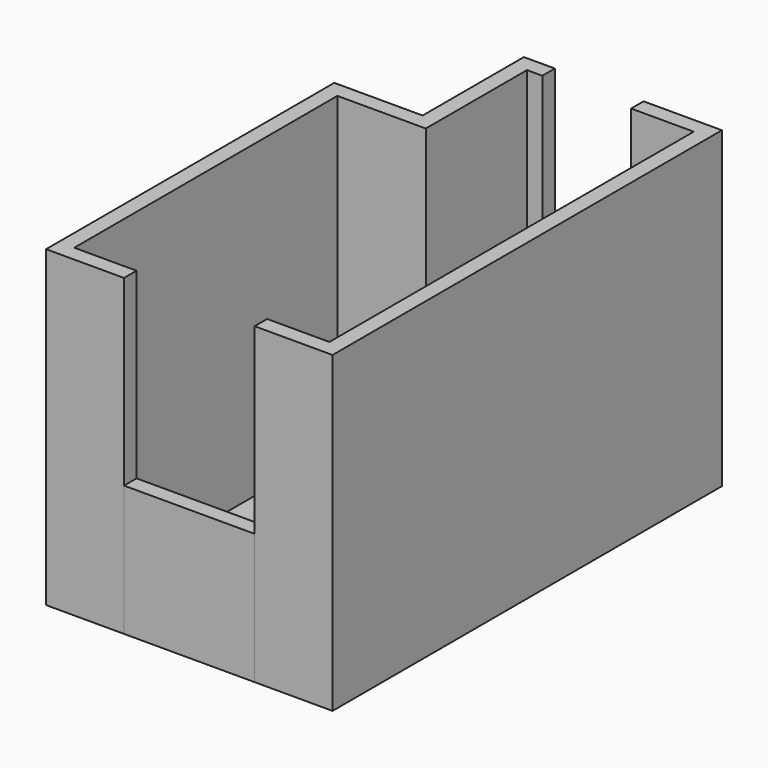
from build123d import *

# Parameters (mm, degrees)
F1_DEPTH = 2400
F0_W     = 1000
F0_H     = 120
F2_DEPTH = 1000
F4_DEPTH = 25


# Not quite as in the source:
# - a feature of the source that left no trace in its solid (it failed there, or was rolled back) is left out


with BuildPart() as f1:
    # F0 (on Top) → F1 (new body)
    with BuildSketch(Plane.XY):
        Polygon((1954, 0), (1477, 0), (1477, -120), (2074, -120), (2074, 3608), (1474, 3608), (1474, 3488), (1954, 3488), align=None)
    extrude(amount=F1_DEPTH)


with BuildPart() as f1b:
    # F0 (on Top) → F1, piece 2 (new body)
    with BuildSketch(Plane.XY):
        Polygon((398.1228470802, 0), (0, 0), (0, 2519), (677, 2519), (677, 3488), (794, 3488), (794, 3608), (677, 3608), (557, 3608), (557, 2639), (-120, 2639), (-120, 2519), (-120, -120), (398.1228470802, -120), (477, -120), (477, 0), align=None)
    extrude(amount=F1_DEPTH)


with BuildPart() as f2:
    # F0 (on Top) → F2 (new body)
    with BuildSketch(Plane.XY):
        with Locations((977, -60)):
            Rectangle(F0_W, F0_H)
    extrude(amount=F2_DEPTH)


with BuildPart() as f4:
    # F0 (on Top) → F4 (new body)
    with BuildSketch(Plane.XY):
        with BuildLine():
            Line((0, 2519), (0, 0))
            Line((0, 0), (398.1228470802, 0))
            Line((398.1228470802, 0), (477, 0))
            Line((477, 0), (1477, 0))
            Line((1477, 0), (1954, 0))
            Line((1954, 0), (1954, 3488))
            Line((1954, 3488), (1474, 3488))
            ThreePointArc((1474, 3488), (1274.8326112069, 3007.1673887931), (794, 2808))
            Line((794, 2808), (794, 3488))
            Line((794, 3488), (677, 3488))
            Line((677, 3488), (677, 2519))
            Line((677, 2519), (0, 2519))
        make_face()
    extrude(amount=F4_DEPTH)


solid = Compound([f1.part, f1b.part, f2.part, f4.part])
